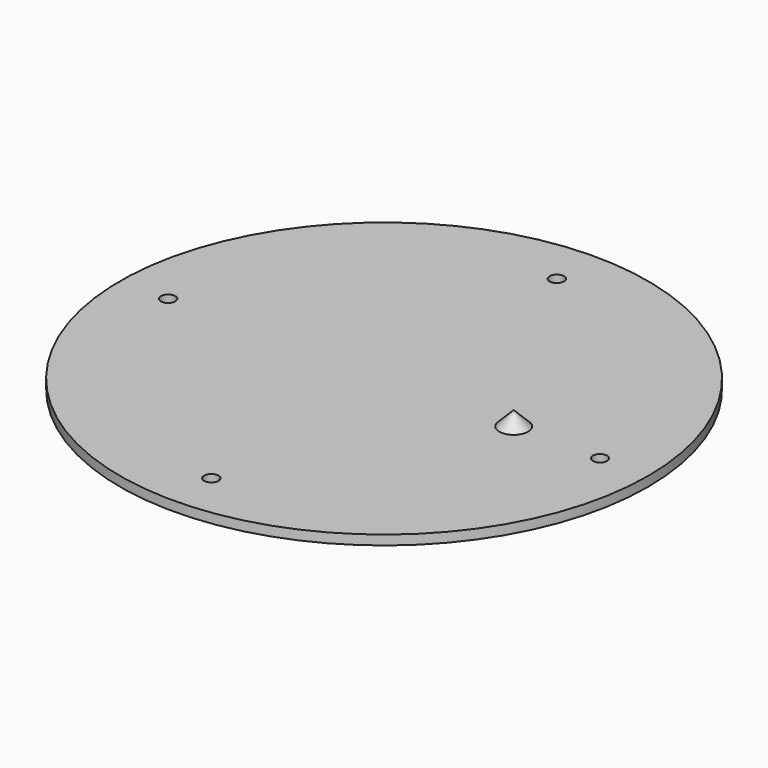
from build123d import *

# Parameters (mm, degrees)
F0_R     = 55
F1_DEPTH = 2
F2_R     = 1.5
F3_DEPTH = 25
F4_R     = 5
F5_DEPTH = 3


# Not quite as in the source:
# - a fillet or chamfer that OpenCascade refuses, or shapes differently, is made with other operations: its cross-section is extruded or revolved along the edge and cut away or added
# - a feature names something its author has since deleted; it is built from what else it names


with BuildPart() as f1:
    # F0 (on Top) → F1 (new body)
    with BuildSketch(Plane.XY):
        Circle(F0_R)
    extrude(amount=F1_DEPTH)

    # F2 (on face) → F3 (cut)
    with BuildSketch(Plane(origin=(0, 0, 0), x_dir=(1, 0, 0), z_dir=(0, 0, -1))):
        with Locations((-45, 0)):
            Circle(F2_R)
        with Locations((0, 45)):
            Circle(F2_R)
        with Locations((45, 0)):
            Circle(F2_R)
        with Locations((0, -45)):
            Circle(F2_R)
    extrude(amount=-F3_DEPTH, mode=Mode.SUBTRACT)

    # F4 (on face) → F5 (join)
    with BuildSketch(Plane.XY.offset(2)):
        with Locations((27, 0)):
            Circle(F4_R)
    extrude(amount=F5_DEPTH)

    # F6: chamfer of 5 on 1 edges, made by hand


with BuildPart() as f6_tool2:
    # F6_s3 → F6_t4 (revolve)
    with BuildSketch(Plane.XZ):
        Polygon((32, 0), (27, 5), (32, 5), align=None)
    revolve(axis=Axis((27, 0, 5), (0, 0, 1)))

    split(bisect_by=Plane.XY.offset(2), keep=Keep.TOP)


with BuildPart() as f1_1:
    add(f1.part)

    # F6_t1: cut F6_tool2
    add(f6_tool2.part, mode=Mode.SUBTRACT)


solid = f1_1.part
